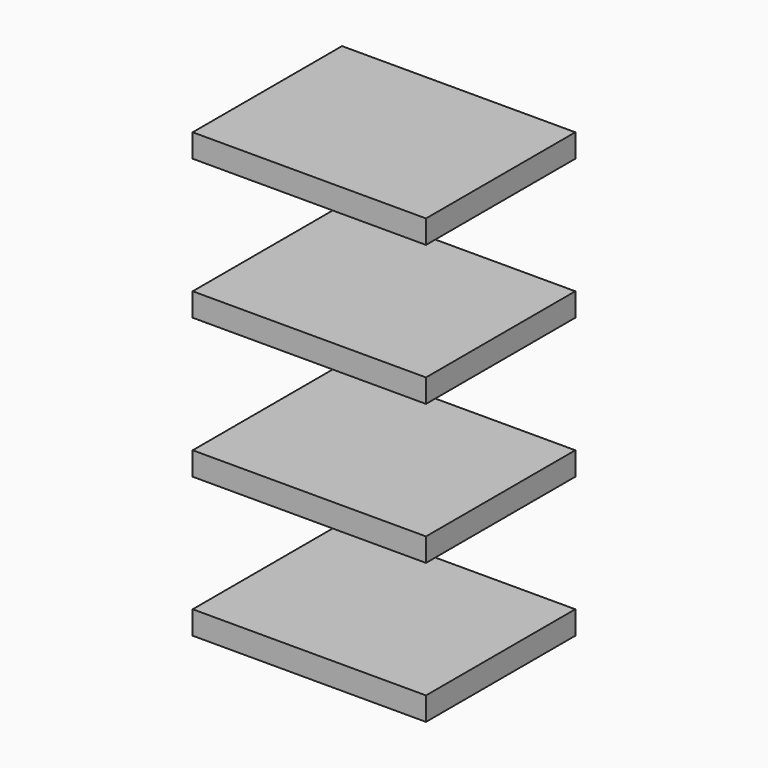
from build123d import *

# Parameters (mm, degrees)
F0_W     = 127
F0_H     = 12.7
F1_DEPTH = 50.8


# Not quite as in the source:
# - the program builds the solid bodies; features that only make, move or delete a surface that nothing else refers to are left out


with BuildPart() as f1:
    # F0 (on Front) → F1 (new body, symmetric)
    with BuildSketch(Plane.XZ):
        with Locations((0, 76.2)):
            Rectangle(F0_W, F0_H)
    extrude(amount=F1_DEPTH, both=True)


with BuildPart() as f1b:
    # F0 (on Front) → F1, piece 2 (new body, symmetric)
    with BuildSketch(Plane.XZ):
        Rectangle(F0_W, F0_H)
    extrude(amount=F1_DEPTH, both=True)


with BuildPart() as f1c:
    # F0 (on Front) → F1, piece 3 (new body, symmetric)
    with BuildSketch(Plane.XZ):
        with Locations((0, -76.2)):
            Rectangle(F0_W, F0_H)
    extrude(amount=F1_DEPTH, both=True)


with BuildPart() as f1d:
    # F0 (on Front) → F1, piece 4 (new body, symmetric)
    with BuildSketch(Plane.XZ):
        with Locations((0, -152.4)):
            Rectangle(F0_W, F0_H)
    extrude(amount=F1_DEPTH, both=True)


solid = Compound([f1.part, f1b.part, f1c.part, f1d.part])
